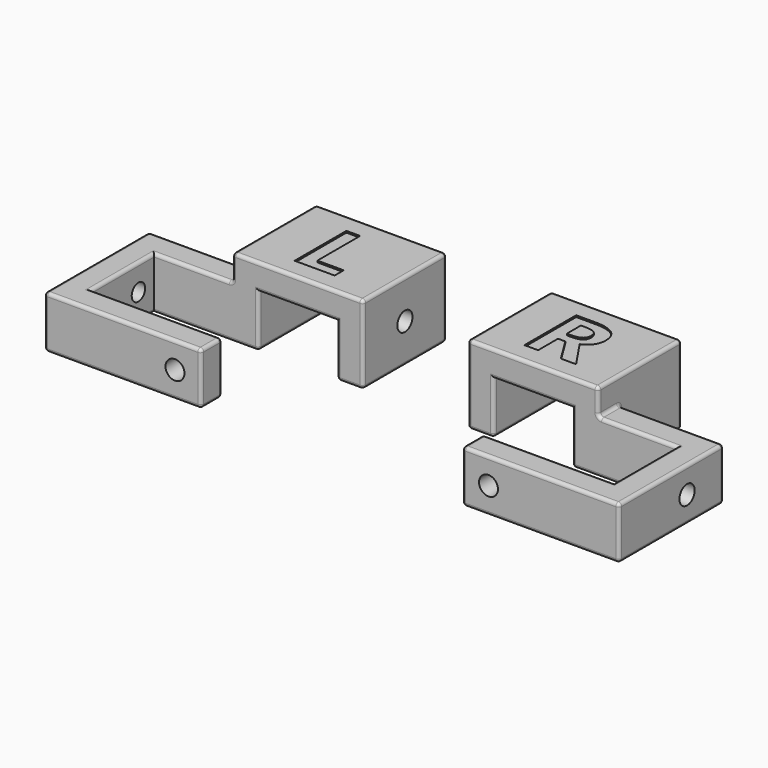
from build123d import *

# Parameters (mm, degrees)
F1_DEPTH      = 25.4
F2_W          = 63.5
F2_H          = 50.8
F3_DEPTH      = 12.7
F4_W          = 12.7
F4_H          = 50.8
F5_DEPTH      = 25.4
F10_R         = 4.6101
F11_R         = 4.0767
F6_R          = 4.6101
F7_R          = 4.0767
F8_R          = 4.6101
F9_R          = 4.0767
F15_R         = 1.5875
F18_TEXT_SIZE = 44.0972222222
F19_TEXT_SIZE = 44.0972222222
F20_DEPTH     = 0.79375


# Not quite as in the source:
# - Text() gives the source's letters only with a copy of the font that has no kerning and outlines rounded to 1/6400 em; it was checked with that copy


with BuildPart() as f1:
    # F0 (on Top) → F1 (new body)
    with BuildSketch(Plane.XY):
        Polygon((-75.6953790172, -16.27197957), (0.5046209828, -16.27197957), (0.5046209828, -3.57197957), (-62.9953790172, -3.57197957), (-62.9953790172, 34.52802043), (-12.1953790172, 34.52802043), (-12.1953790172, 85.32802043), (-24.8953790172, 85.32802043), (-24.8953790172, 47.22802043), (-75.6953790172, 47.22802043), align=None)
    extrude(amount=F1_DEPTH)

    # F2 (on face) → F3 (join)
    with BuildSketch(Plane.XY.offset(25.4)):
        with Locations((6.8546209828, 59.92802043)):
            Rectangle(F2_W, F2_H)
    extrude(amount=F3_DEPTH)

    # F4 (on face) → F5 (join)
    with BuildSketch(Plane(origin=(0, 0, 25.4), x_dir=(1, 0, 0), z_dir=(0, 0, -1))):
        with Locations((32.2546209828, -59.92802043)):
            Rectangle(F4_W, F4_H)
    extrude(amount=F5_DEPTH)

    # F10 (on face) → F12 section 0
    with BuildSketch(Plane.YZ.offset(38.6046209828)):
        with Locations((59.92802043, 19.05)):
            Circle(F10_R)
    # F11 (on face) → F12 section 1
    with BuildSketch(Plane(origin=(25.9046209828, 0, 0), x_dir=(0, -1, 0), z_dir=(-1, 0, 0))):
        with Locations((-59.92802043, 19.05)):
            Circle(F11_R)
    loft(mode=Mode.SUBTRACT)

    # F6 (on face) → F13 section 0
    with BuildSketch(Plane.XZ.offset(16.27197957)):
        with Locations((-12.1953790172, 12.7)):
            Circle(F6_R)
    # F7 (on face) → F13 section 1
    with BuildSketch(Plane(origin=(0, -3.57197957, 0), x_dir=(-1, 0, 0), z_dir=(0, 1, 0))):
        with Locations((12.1953790172, 12.7)):
            Circle(F7_R)
    loft(mode=Mode.SUBTRACT)

    # F8 (on face) → F14 section 0
    with BuildSketch(Plane(origin=(-75.6953790172, 0, 0), x_dir=(0, -1, 0), z_dir=(-1, 0, 0))):
        with Locations((-25.00302043, 12.7)):
            Circle(F8_R)
    # F9 (on face) → F14 section 1
    with BuildSketch(Plane.YZ.offset(-62.9953790172)):
        with Locations((25.00302043, 12.7)):
            Circle(F9_R)
    loft(mode=Mode.SUBTRACT)

    # F15
    f15_edges = [f1.edges().sort_by_distance(p)[0] for p in [
        (-24.895379, 40.87802, 25.4),
        (-43.945379, 34.52802, 25.4),
        (-62.995379, 15.47802, 25.4),
        (-31.245379, -3.57198, 25.4),
        (0.504621, -9.92198, 25.4),
        (-37.595379, -16.27198, 25.4),
        (-75.695379, 15.47802, 25.4),
        (-50.295379, 47.22802, 25.4),
        (-50.295379, 47.22802, 0),
        (-75.695379, 15.47802, 0),
        (-37.595379, -16.27198, 0),
        (0.504621, -9.92198, 0),
        (-31.245379, -3.57198, 0),
        (-62.995379, 15.47802, 0),
        (-37.595379, 34.52802, 0),
        (-12.195379, 59.92802, 0),
        (-18.545379, 85.32802, 0),
        (-24.895379, 66.27802, 0),
        (38.604621, 59.92802, 0),
        (32.254621, 34.52802, 0),
        (25.904621, 59.92802, 0),
        (32.254621, 85.32802, 0),
        (-12.195379, 85.32802, 12.7),
        (6.854621, 85.32802, 25.4),
        (25.904621, 85.32802, 12.7),
        (38.604621, 85.32802, 19.05),
        (6.854621, 85.32802, 38.1),
        (-24.895379, 85.32802, 19.05),
        (-24.895379, 59.92802, 38.1),
        (-24.895379, 34.52802, 31.75),
        (-24.895379, 47.22802, 12.7),
        (38.604621, 59.92802, 38.1),
        (6.854621, 34.52802, 38.1),
        (0.504621, -16.27198, 12.7),
        (0.504621, -3.57198, 12.7),
        (38.604621, 34.52802, 19.05),
        (25.904621, 34.52802, 12.7),
        (6.854621, 34.52802, 25.4),
        (-12.195379, 34.52802, 12.7),
        (-75.695379, -16.27198, 12.7),
        (-75.695379, 47.22802, 12.7),
    ]]
    fillet(f15_edges, radius=F15_R)


with BuildPart() as f17_1:
    # F17: instance of F1
    add(f1.part.mirror(Plane(origin=(64.0046209828, 59.92802043, 19.05), x_dir=(0, 1, 0), z_dir=(1, 0, 0))))


with BuildPart() as f20_tool:
    # F18 (on face) + F19 (on face) → F20 (new body)
    with BuildSketch(Plane.XY.offset(38.1)):
        with Locations((-6.2780830103, 44.05302043)):
            Text('L', F18_TEXT_SIZE, font='Open Sans', font_style=FontStyle.BOLD, text_align=(TextAlign.LEFT, TextAlign.BOTTOM))
    with BuildSketch(Plane.XY.offset(38.1)):
        with Locations((105.1693779272, 44.3709143847)):
            Text('R', F19_TEXT_SIZE, font='Open Sans', font_style=FontStyle.BOLD, text_align=(TextAlign.LEFT, TextAlign.BOTTOM))
    extrude(amount=-F20_DEPTH)


with BuildPart() as f1_1:
    add(f1.part)

    # F20: cut by f20_tool
    add(f20_tool.part, mode=Mode.SUBTRACT)


with BuildPart() as f17_1_1:
    add(f17_1.part)

    # F20: cut by f20_tool
    add(f20_tool.part, mode=Mode.SUBTRACT)


solid = Compound([f1_1.part, f17_1_1.part])
